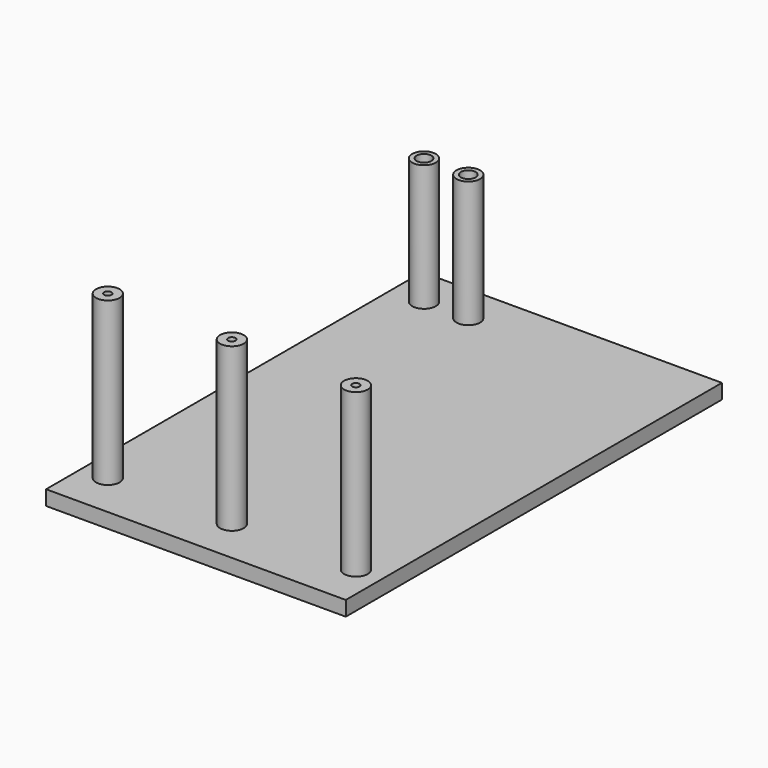
from build123d import *

# Parameters (mm, degrees)
F0_W            = 64.4398
F0_H            = 104.267
F1_DEPTH        = 3.175
F2_W            = 64.4398
F2_H            = 3.175
F3_DEPTH        = 34.925
F4_R            = 1.5875
F5_DEPTH        = 3.176
F6_R            = 2.54
F6_R_2          = 1.5875
F7_DEPTH        = 27.178
F8_W            = 1.016
F8_H            = 38.1
F9_DEPTH        = 1.5875
F10_W           = 1.016
F10_H           = 38.1
F11_DEPTH       = 1.5875
F12_R           = 1.524
F13_DEPTH       = 3.175
F14_TEXT_SIZE   = 3.832154644
F14_TEXT_SIZE_2 = 3.4384220824
F15_DEPTH       = 1.524
F16_W           = 67.6148
F16_H           = 3.175
F17_DEPTH       = 38.1010001
F18_R           = 2.54
F19_DEPTH       = 34.925
F20_R           = 0.79375
F21_DEPTH       = 12.7


# Not quite as in the source:
# - Text() gives the source's letters only with a copy of the font that has no kerning and outlines rounded to 1/6400 em; it was checked with that copy


with BuildPart() as f1:
    # F0 (on Top) → F1 (new body)
    with BuildSketch(Plane.XY):
        with Locations((-32.2199, 52.1335)):
            Rectangle(F0_W, F0_H)
    extrude(amount=F1_DEPTH)

    # F2 (on face) → F3 (join)
    with BuildSketch(Plane.XY.offset(3.175)):
        with Locations((-32.2199, 1.5875)):
            Rectangle(F2_W, F2_H)
    extrude(amount=F3_DEPTH)

    # F4 (on face) → F5 (cut, through all)
    with BuildSketch(Plane.XY.offset(3.175)):
        with Locations((-57.4548, 96.012)):
            Circle(F4_R)
        with Locations((-47.9298, 96.012)):
            Circle(F4_R)
    extrude(amount=-F5_DEPTH, mode=Mode.SUBTRACT)

    # F6 (on face) → F7 (join)
    with BuildSketch(Plane.XY.offset(3.175)):
        with Locations((-57.4548, 96.012)):
            Circle(F6_R)
        with Locations((-57.4548, 96.012)):
            Circle(F6_R_2, mode=Mode.SUBTRACT)
        with Locations((-47.9298, 96.012)):
            Circle(F6_R)
        with Locations((-47.9298, 96.012)):
            Circle(F6_R_2, mode=Mode.SUBTRACT)
    extrude(amount=F7_DEPTH)

    # F8 (on face) → F9 (join)
    with BuildSketch(Plane.YZ):
        with Locations((2.667, 19.05)):
            Rectangle(F8_W, F8_H)
    extrude(amount=F9_DEPTH)

    # F10 (on face) → F11 (join)
    with BuildSketch(Plane(origin=(-64.4398, 0, 0), x_dir=(0, -1, 0), z_dir=(-1, 0, 0))):
        with Locations((-2.667, 19.05)):
            Rectangle(F10_W, F10_H)
    extrude(amount=F11_DEPTH)

    # F12 (on face) → F13 (cut, through all)
    with BuildSketch(Plane.XZ):
        Polygon((-24.8158, 4.699), (-5.0038, 4.699), (-6.4008, 15.5312885394), (-23.4188, 15.5312885394), align=None)
        Polygon((-24.8158, 26.3973557303), (-5.0038, 26.3973557303), (-6.4008, 37.2296442697), (-23.4188, 37.2296442697), align=None)
        Polygon((-59.436, 4.699), (-39.624, 4.699), (-41.021, 15.5312885394), (-58.039, 15.5312885394), align=None)
        Polygon((-59.436, 26.3973557303), (-39.624, 26.3973557303), (-41.021, 37.2296442697), (-58.039, 37.2296442697), align=None)
        with Locations((-27.6098, 10.1151442697)):
            Circle(F12_R)
        with Locations((-2.2098, 10.1151442697)):
            Circle(F12_R)
        with Locations((-2.2098, 31.8135)):
            Circle(F12_R)
        with Locations((-27.6098, 31.8135)):
            Circle(F12_R)
        with Locations((-36.83, 31.8135)):
            Circle(F12_R)
        with Locations((-62.23, 31.8135)):
            Circle(F12_R)
        with Locations((-62.23, 10.1151442697)):
            Circle(F12_R)
        with Locations((-36.83, 10.1151442697)):
            Circle(F12_R)
    extrude(amount=-F13_DEPTH, mode=Mode.SUBTRACT)

    # F14 (on face) → F15 (cut)
    with BuildSketch(Plane(origin=(0, 0, 0), x_dir=(1, 0, 0), z_dir=(0, 0, -1))):
        with Locations(Location((-44.1827221612, -91.7315941418), (0, 0, 90))):
            Text('PWR', F14_TEXT_SIZE, font='Open Sans', font_style=FontStyle.BOLD, text_align=(TextAlign.LEFT, TextAlign.BOTTOM))
        with Locations(Location((-53.0572757125, -91.7315941418), (0, 0, 90))):
            Text('RESET', F14_TEXT_SIZE_2, font='Open Sans', font_style=FontStyle.BOLD, text_align=(TextAlign.LEFT, TextAlign.BOTTOM))
    extrude(amount=-F15_DEPTH, mode=Mode.SUBTRACT)

    # F16 (on face) → F17 (cut, through all)
    with BuildSketch(Plane.XY.offset(38.1)):
        with Locations((-32.2199, 1.5875)):
            Rectangle(F16_W, F16_H)
    extrude(amount=-F17_DEPTH, mode=Mode.SUBTRACT)

    # F18 (on face) → F19 (join)
    with BuildSketch(Plane.XY.offset(3.175)):
        with Locations((-32.2199, 12.827)):
            Circle(F18_R)
        with Locations((-58.8899, 12.827)):
            Circle(F18_R)
        with Locations((-5.5499, 12.827)):
            Circle(F18_R)
    extrude(amount=F19_DEPTH)

    # F20 (on face) → F21 (cut)
    with BuildSketch(Plane.XY.offset(38.1)):
        with Locations((-5.5499, 12.827)):
            Circle(F20_R)
        with Locations((-32.2199, 12.827)):
            Circle(F20_R)
        with Locations((-58.8899, 12.827)):
            Circle(F20_R)
    extrude(amount=-F21_DEPTH, mode=Mode.SUBTRACT)


solid = f1.part
